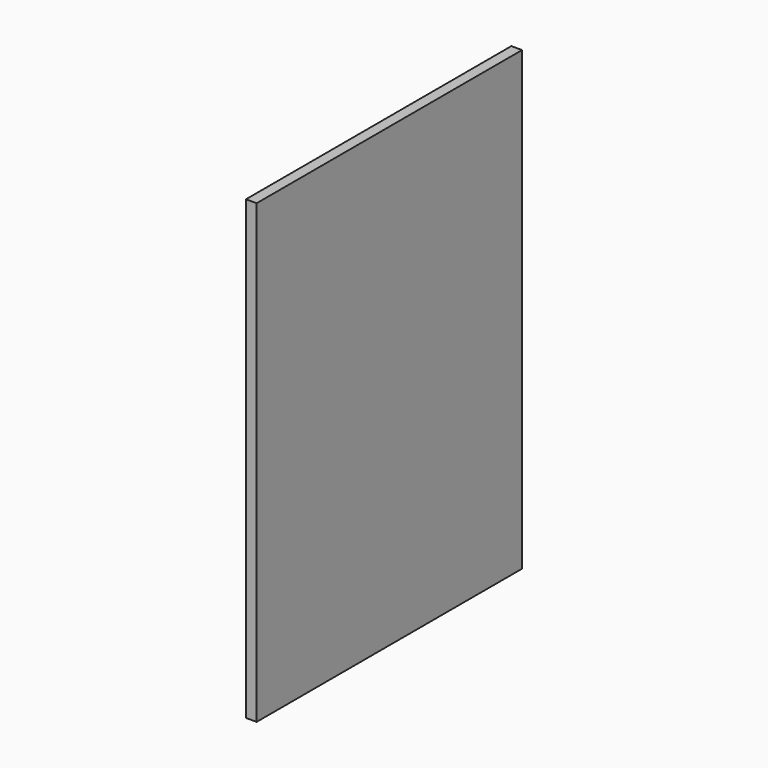
from build123d import *

# Parameters (mm, degrees)
F0_W     = 4.65
F0_H     = 6.4
F1_DEPTH = 0.15
F3_DEPTH = 0.2
F4_R     = 0.19999
F4_2_R   = 0.19999
F4_3_R   = 0.19999
F4_4_R   = 0.19999


# Not quite as in the source:
# - a fillet or chamfer is up to 0.001 mm smaller than in the source, because OpenCascade refuses the exact size


with BuildPart() as f1:
    # F0 (on Right) → F1 (new body)
    with BuildSketch(Plane.YZ):
        with Locations((0, 3.2)):
            Rectangle(F0_W, F0_H)
    extrude(amount=-F1_DEPTH)


with BuildPart() as f3:
    # F2 (on face) → F3 (new body)
    with BuildSketch(Plane(origin=(-0.15, 0, 0), x_dir=(0, -1, 0), z_dir=(-1, 0, 0))):
        with BuildLine():
            Line((-1.55, 0.45), (1.55, 0.45))
            ThreePointArc((1.55, 0.45), (1.7267766953, 0.5232233047), (1.8, 0.7))
            Line((1.8, 0.7), (1.8, 1.2))
            ThreePointArc((1.8, 1.2), (1.7267766953, 1.3767766953), (1.55, 1.45))
            Line((1.55, 1.45), (-1.55, 1.45))
            ThreePointArc((-1.55, 1.45), (-1.7267766953, 1.3767766953), (-1.8, 1.2))
            Line((-1.8, 1.2), (-1.8, 0.7))
            ThreePointArc((-1.8, 0.7), (-1.7267766953, 0.5232233047), (-1.55, 0.45))
        make_face()
    extrude(amount=F3_DEPTH)

    # F4#4 (radius 0.2 in the source; OpenCascade refuses exactly that, so slightly less here)
    f4_4_edges = [f3.edges().sort_by_distance(p)[0] for p in [
        (-0.35, 0, 0.45),
        (-0.35, -1.726777, 0.523223),
        (-0.35, -1.8, 0.95),
        (-0.35, -1.726777, 1.376777),
        (-0.35, 0, 1.45),
        (-0.35, 1.726777, 1.376777),
        (-0.35, 1.8, 0.95),
        (-0.35, 1.726777, 0.523223),
    ]]
    fillet(f4_4_edges, radius=F4_4_R)


with BuildPart() as f3b:
    # F2 (on face) → F3, piece 2 (new body)
    with BuildSketch(Plane(origin=(-0.15, 0, 0), x_dir=(0, -1, 0), z_dir=(-1, 0, 0))):
        with BuildLine():
            Line((-1.5452531883, 1.9499924892), (1.5547468117, 1.9499924892))
            ThreePointArc((1.5547468117, 1.9499924892), (1.731523507, 2.0232157939), (1.8047468117, 2.1999924892))
            Line((1.8047468117, 2.1999924892), (1.8047468117, 2.6999924892))
            ThreePointArc((1.8047468117, 2.6999924892), (1.731523507, 2.8767691845), (1.5547468117, 2.9499924892))
            Line((1.5547468117, 2.9499924892), (-1.5452531883, 2.9499924892))
            ThreePointArc((-1.5452531883, 2.9499924892), (-1.7220298836, 2.8767691845), (-1.7952531883, 2.6999924892))
            Line((-1.7952531883, 2.6999924892), (-1.7952531883, 2.1999924892))
            ThreePointArc((-1.7952531883, 2.1999924892), (-1.7220298836, 2.0232157939), (-1.5452531883, 1.9499924892))
        make_face()
    extrude(amount=F3_DEPTH)

    # F4#3 (radius 0.2 in the source; OpenCascade refuses exactly that, so slightly less here)
    f4_3_edges = [f3b.edges().sort_by_distance(p)[0] for p in [
        (-0.35, 1.72203, 2.023216),
        (-0.35, -0.004747, 1.949992),
        (-0.35, -1.731524, 2.023216),
        (-0.35, -1.804747, 2.449992),
        (-0.35, -1.731524, 2.876769),
        (-0.35, -0.004747, 2.949992),
        (-0.35, 1.72203, 2.876769),
        (-0.35, 1.795253, 2.449992),
    ]]
    fillet(f4_3_edges, radius=F4_3_R)


with BuildPart() as f3c:
    # F2 (on face) → F3, piece 3 (new body)
    with BuildSketch(Plane(origin=(-0.15, 0, 0), x_dir=(0, -1, 0), z_dir=(-1, 0, 0))):
        with BuildLine():
            Line((-1.5405063767, 3.4499849785), (1.5594936233, 3.4499849785))
            ThreePointArc((1.5594936233, 3.4499849785), (1.7362703186, 3.5232082832), (1.8094936233, 3.6999849785))
            Line((1.8094936233, 3.6999849785), (1.8094936233, 4.1999849785))
            ThreePointArc((1.8094936233, 4.1999849785), (1.7362703186, 4.3767616738), (1.5594936233, 4.4499849785))
            Line((1.5594936233, 4.4499849785), (-1.5405063767, 4.4499849785))
            ThreePointArc((-1.5405063767, 4.4499849785), (-1.7172830719, 4.3767616738), (-1.7905063767, 4.1999849785))
            Line((-1.7905063767, 4.1999849785), (-1.7905063767, 3.6999849785))
            ThreePointArc((-1.7905063767, 3.6999849785), (-1.7172830719, 3.5232082832), (-1.5405063767, 3.4499849785))
        make_face()
    extrude(amount=F3_DEPTH)

    # F4#2 (radius 0.2 in the source; OpenCascade refuses exactly that, so slightly less here)
    f4_2_edges = [f3c.edges().sort_by_distance(p)[0] for p in [
        (-0.35, 1.717283, 3.523208),
        (-0.35, -0.009494, 3.449985),
        (-0.35, -1.73627, 3.523208),
        (-0.35, -1.809494, 3.949985),
        (-0.35, -1.73627, 4.376762),
        (-0.35, -0.009494, 4.449985),
        (-0.35, 1.717283, 4.376762),
        (-0.35, 1.790506, 3.949985),
    ]]
    fillet(f4_2_edges, radius=F4_2_R)


with BuildPart() as f3d:
    # F2 (on face) → F3, piece 4 (new body)
    with BuildSketch(Plane(origin=(-0.15, 0, 0), x_dir=(0, -1, 0), z_dir=(-1, 0, 0))):
        with BuildLine():
            Line((-1.535759565, 4.9499774677), (1.564240435, 4.9499774677))
            ThreePointArc((1.564240435, 4.9499774677), (1.7410171303, 5.0232007724), (1.814240435, 5.1999774677))
            Line((1.814240435, 5.1999774677), (1.814240435, 5.6999774677))
            ThreePointArc((1.814240435, 5.6999774677), (1.7410171303, 5.876754163), (1.564240435, 5.9499774677))
            Line((1.564240435, 5.9499774677), (-1.535759565, 5.9499774677))
            ThreePointArc((-1.535759565, 5.9499774677), (-1.7125362603, 5.876754163), (-1.785759565, 5.6999774677))
            Line((-1.785759565, 5.6999774677), (-1.785759565, 5.1999774677))
            ThreePointArc((-1.785759565, 5.1999774677), (-1.7125362603, 5.0232007724), (-1.535759565, 4.9499774677))
        make_face()
    extrude(amount=F3_DEPTH)

    # F4 (radius 0.2 in the source; OpenCascade refuses exactly that, so slightly less here)
    f4_edges = [f3d.edges().sort_by_distance(p)[0] for p in [
        (-0.35, 1.712536, 5.023201),
        (-0.35, -0.01424, 4.949977),
        (-0.35, -1.741017, 5.023201),
        (-0.35, -1.81424, 5.449977),
        (-0.35, -1.741017, 5.876754),
        (-0.35, -0.01424, 5.949977),
        (-0.35, 1.712536, 5.876754),
        (-0.35, 1.78576, 5.449977),
    ]]
    fillet(f4_edges, radius=F4_R)


solid = Compound([f1.part, f3.part, f3b.part, f3c.part, f3d.part])
